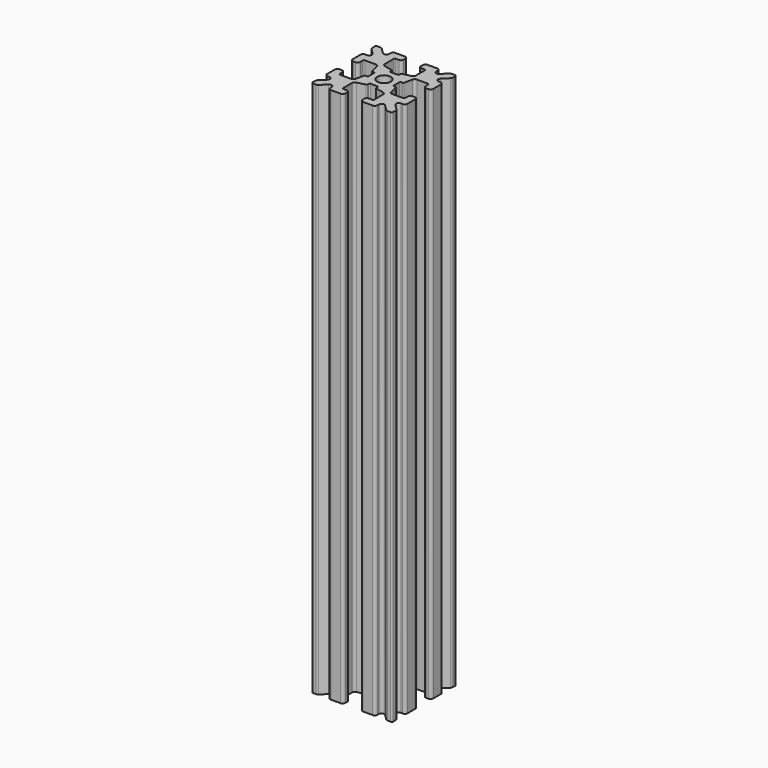
from build123d import *

# Parameters (mm, degrees)
F0_R     = 1.25
F1_DEPTH = 100


# Not quite as in the source:
# - ends of sketch curves that miss each other by under 0.0002 mm in the source are joined


with BuildPart() as f1:
    # F0 (on Top) → F1 (new body)
    with BuildSketch(Plane.XY):
        with BuildLine():
            Line((-0.6255, -2.347065), (0.6255, -2.347065))
            ThreePointArc((0.6255, -2.347065), (0.7669213562, -2.4056436438), (0.8255, -2.547065))
            Line((0.8255, -2.547065), (0.8255, -2.774891))
            ThreePointArc((0.8255, -2.774891), (0.8693776134, -2.8998942016), (0.9817580041, -2.9700489816))
            Line((0.9817580041, -2.9700489816), (2.509356, -3.312442))
            ThreePointArc((2.509356, -3.312442), (2.7903062714, -3.4878293768), (2.9, -3.800337))
            Line((2.9, -3.800337), (2.9, -5.9))
            ThreePointArc((2.9, -5.9), (2.8414213562, -6.0414213562), (2.7, -6.1))
            Line((2.7, -6.1), (2.1, -6.1))
            ThreePointArc((2.1, -6.1), (1.7464466094, -6.2464466094), (1.6, -6.6))
            Line((1.6, -6.6), (1.6, -7))
            ThreePointArc((1.6, -7), (1.7464466094, -7.3535533906), (2.1, -7.5))
            Line((2.1, -7.5), (3.9, -7.5))
            ThreePointArc((3.9, -7.5), (4.2535533906, -7.3535533906), (4.4, -7))
            Line((4.4, -7), (4.4, -6.667767))
            ThreePointArc((4.4, -6.667767), (4.7086582838, -6.2058272337), (5.2535533906, -6.3142136094))
            Line((5.2535533906, -6.3142136094), (6.292893, -7.353553))
            ThreePointArc((6.292893, -7.353553), (6.4551049572, -7.461939631), (6.646447, -7.5))
            Line((6.646447, -7.5), (7.25, -7.5))
            ThreePointArc((7.25, -7.5), (7.4267766953, -7.4267766953), (7.5, -7.25))
            Line((7.5, -7.25), (7.5, -6.646447))
            ThreePointArc((7.5, -6.646447), (7.461939631, -6.4551049572), (7.3535528906, -6.2928931094))
            Line((7.3535528906, -6.2928931094), (6.314214, -5.253553))
            ThreePointArc((6.314214, -5.253553), (6.2058272337, -4.7086582838), (6.667767, -4.4))
            Line((6.667767, -4.4), (7, -4.4))
            ThreePointArc((7, -4.4), (7.3535533906, -4.2535533906), (7.5, -3.9))
            Line((7.5, -3.9), (7.5, -2.1))
            ThreePointArc((7.5, -2.1), (7.3535533906, -1.7464466094), (7, -1.6))
            Line((7, -1.6), (6.6, -1.6))
            ThreePointArc((6.6, -1.6), (6.2464466094, -1.7464466094), (6.1, -2.1))
            Line((6.1, -2.1), (6.1, -2.7))
            ThreePointArc((6.1, -2.7), (6.0414213562, -2.8414213562), (5.9, -2.9))
            Line((5.9, -2.9), (3.800337, -2.9))
            ThreePointArc((3.800337, -2.9), (3.4878293768, -2.7903062714), (3.3124422593, -2.5093559419))
            Line((3.3124422593, -2.5093559419), (2.970049, -0.981758))
            ThreePointArc((2.970049, -0.981758), (2.8998942016, -0.8693776134), (2.774891, -0.8255))
            Line((2.774891, -0.8255), (2.547065, -0.8255))
            ThreePointArc((2.547065, -0.8255), (2.4056436438, -0.7669213562), (2.347065, -0.6255))
            Line((2.347065, -0.6255), (2.347065, 0.6255))
            ThreePointArc((2.347065, 0.6255), (2.4056436438, 0.7669213562), (2.547065, 0.8255))
            Line((2.547065, 0.8255), (2.774891, 0.8255))
            ThreePointArc((2.774891, 0.8255), (2.8998942016, 0.8693776134), (2.9700489816, 0.9817580041))
            Line((2.9700489816, 0.9817580041), (3.312442, 2.509356))
            ThreePointArc((3.312442, 2.509356), (3.4878293768, 2.7903062714), (3.800337, 2.9))
            Line((3.800337, 2.9), (5.9, 2.9))
            ThreePointArc((5.9, 2.9), (6.0414213562, 2.8414213562), (6.1, 2.7))
            Line((6.1, 2.7), (6.1, 2.1))
            ThreePointArc((6.1, 2.1), (6.2464466094, 1.7464466094), (6.6, 1.6))
            Line((6.6, 1.6), (7, 1.6))
            ThreePointArc((7, 1.6), (7.3535533906, 1.7464466094), (7.5, 2.1))
            Line((7.5, 2.1), (7.5, 3.9))
            ThreePointArc((7.5, 3.9), (7.3535533906, 4.2535533906), (7, 4.4))
            Line((7, 4.4), (6.667767, 4.4))
            ThreePointArc((6.667767, 4.4), (6.2058272337, 4.7086582838), (6.3142136094, 5.2535533906))
            Line((6.3142136094, 5.2535533906), (7.353553, 6.292893))
            ThreePointArc((7.353553, 6.292893), (7.461939631, 6.4551049572), (7.5, 6.646447))
            Line((7.5, 6.646447), (7.5, 7.25))
            ThreePointArc((7.5, 7.25), (7.4267766953, 7.4267766953), (7.25, 7.5))
            Line((7.25, 7.5), (6.646447, 7.5))
            ThreePointArc((6.646447, 7.5), (6.4551049572, 7.461939631), (6.2928931094, 7.3535528906))
            Line((6.2928931094, 7.3535528906), (5.253553, 6.314214))
            ThreePointArc((5.253553, 6.314214), (4.7086582838, 6.2058272337), (4.4, 6.667767))
            Line((4.4, 6.667767), (4.4, 7))
            ThreePointArc((4.4, 7), (4.2535533906, 7.3535533906), (3.9, 7.5))
            Line((3.9, 7.5), (2.1, 7.5))
            ThreePointArc((2.1, 7.5), (1.7464466094, 7.3535533906), (1.6, 7))
            Line((1.6, 7), (1.6, 6.6))
            ThreePointArc((1.6, 6.6), (1.7464466094, 6.2464466094), (2.1, 6.1))
            Line((2.1, 6.1), (2.7, 6.1))
            ThreePointArc((2.7, 6.1), (2.8414213562, 6.0414213562), (2.9, 5.9))
            Line((2.9, 5.9), (2.9, 3.800337))
            ThreePointArc((2.9, 3.800337), (2.7903062714, 3.4878293768), (2.5093559419, 3.3124422593))
            Line((2.5093559419, 3.3124422593), (0.981758, 2.970049))
            ThreePointArc((0.981758, 2.970049), (0.8693776134, 2.8998942016), (0.8255, 2.774891))
            Line((0.8255, 2.774891), (0.8255, 2.547065))
            ThreePointArc((0.8255, 2.547065), (0.7669213562, 2.4056436438), (0.6255, 2.347065))
            Line((0.6255, 2.347065), (-0.6255, 2.347065))
            ThreePointArc((-0.6255, 2.347065), (-0.7669213562, 2.4056436438), (-0.8255, 2.547065))
            Line((-0.8255, 2.547065), (-0.8255, 2.774891))
            ThreePointArc((-0.8255, 2.774891), (-0.8693776134, 2.8998942016), (-0.9817580041, 2.9700489816))
            Line((-0.9817580041, 2.9700489816), (-2.509356, 3.312442))
            ThreePointArc((-2.509356, 3.312442), (-2.7903062714, 3.4878293768), (-2.9, 3.800337))
            Line((-2.9, 3.800337), (-2.9, 5.9))
            ThreePointArc((-2.9, 5.9), (-2.8414213562, 6.0414213562), (-2.7, 6.1))
            Line((-2.7, 6.1), (-2.1, 6.1))
            ThreePointArc((-2.1, 6.1), (-1.7464466094, 6.2464466094), (-1.6, 6.6))
            Line((-1.6, 6.6), (-1.6, 7))
            ThreePointArc((-1.6, 7), (-1.7464466094, 7.3535533906), (-2.1, 7.5))
            Line((-2.1, 7.5), (-3.9, 7.5))
            ThreePointArc((-3.9, 7.5), (-4.2535533906, 7.3535533906), (-4.4, 7))
            Line((-4.4, 7), (-4.4, 6.667767))
            ThreePointArc((-4.4, 6.667767), (-4.7086582838, 6.2058272337), (-5.2535533906, 6.3142136094))
            Line((-5.2535533906, 6.3142136094), (-6.292893, 7.353553))
            ThreePointArc((-6.292893, 7.353553), (-6.4551049572, 7.461939631), (-6.646447, 7.5))
            Line((-6.646447, 7.5), (-7.25, 7.5))
            ThreePointArc((-7.25, 7.5), (-7.4267766953, 7.4267766953), (-7.5, 7.25))
            Line((-7.5, 7.25), (-7.5, 6.646447))
            ThreePointArc((-7.5, 6.646447), (-7.461939631, 6.4551049572), (-7.3535528906, 6.2928931094))
            Line((-7.3535528906, 6.2928931094), (-6.314214, 5.253553))
            ThreePointArc((-6.314214, 5.253553), (-6.2058272337, 4.7086582838), (-6.667767, 4.4))
            Line((-6.667767, 4.4), (-7, 4.4))
            ThreePointArc((-7, 4.4), (-7.3535533906, 4.2535533906), (-7.5, 3.9))
            Line((-7.5, 3.9), (-7.5, 2.1))
            ThreePointArc((-7.5, 2.1), (-7.3535533906, 1.7464466094), (-7, 1.6))
            Line((-7, 1.6), (-6.6, 1.6))
            ThreePointArc((-6.6, 1.6), (-6.2464466094, 1.7464466094), (-6.1, 2.1))
            Line((-6.1, 2.1), (-6.1, 2.7))
            ThreePointArc((-6.1, 2.7), (-6.0414213562, 2.8414213562), (-5.9, 2.9))
            Line((-5.9, 2.9), (-3.800337, 2.9))
            ThreePointArc((-3.800337, 2.9), (-3.4878293768, 2.7903062714), (-3.3124422593, 2.5093559419))
            Line((-3.3124422593, 2.5093559419), (-2.970049, 0.981758))
            ThreePointArc((-2.970049, 0.981758), (-2.8998942016, 0.8693776134), (-2.774891, 0.8255))
            Line((-2.774891, 0.8255), (-2.547065, 0.8255))
            ThreePointArc((-2.547065, 0.8255), (-2.4056436438, 0.7669213562), (-2.347065, 0.6255))
            Line((-2.347065, 0.6255), (-2.347065, -0.6255))
            ThreePointArc((-2.347065, -0.6255), (-2.4056436438, -0.7669213562), (-2.547065, -0.8255))
            Line((-2.547065, -0.8255), (-2.774891, -0.8255))
            ThreePointArc((-2.774891, -0.8255), (-2.8998942016, -0.8693776134), (-2.9700489816, -0.9817580041))
            Line((-2.9700489816, -0.9817580041), (-3.312442, -2.509356))
            ThreePointArc((-3.312442, -2.509356), (-3.4878293768, -2.7903062714), (-3.800337, -2.9))
            Line((-3.800337, -2.9), (-5.9, -2.9))
            ThreePointArc((-5.9, -2.9), (-6.0414213562, -2.8414213562), (-6.1, -2.7))
            Line((-6.1, -2.7), (-6.1, -2.1))
            ThreePointArc((-6.1, -2.1), (-6.2464466094, -1.7464466094), (-6.6, -1.6))
            Line((-6.6, -1.6), (-7, -1.6))
            ThreePointArc((-7, -1.6), (-7.3535533906, -1.7464466094), (-7.5, -2.1))
            Line((-7.5, -2.1), (-7.5, -3.9))
            ThreePointArc((-7.5, -3.9), (-7.3535533906, -4.2535533906), (-7, -4.4))
            Line((-7, -4.4), (-6.667767, -4.4))
            ThreePointArc((-6.667767, -4.4), (-6.2058272337, -4.7086582838), (-6.3142136094, -5.2535533906))
            Line((-6.3142136094, -5.2535533906), (-7.353553, -6.292893))
            ThreePointArc((-7.353553, -6.292893), (-7.461939631, -6.4551049572), (-7.5, -6.646447))
            Line((-7.5, -6.646447), (-7.5, -7.25))
            ThreePointArc((-7.5, -7.25), (-7.4267766953, -7.4267766953), (-7.25, -7.5))
            Line((-7.25, -7.5), (-6.646447, -7.5))
            ThreePointArc((-6.646447, -7.5), (-6.4551049572, -7.461939631), (-6.2928931094, -7.3535528906))
            Line((-6.2928931094, -7.3535528906), (-5.253553, -6.314214))
            ThreePointArc((-5.253553, -6.314214), (-4.7086582838, -6.2058272337), (-4.4, -6.667767))
            Line((-4.4, -6.667767), (-4.4, -7))
            ThreePointArc((-4.4, -7), (-4.2535533906, -7.3535533906), (-3.9, -7.5))
            Line((-3.9, -7.5), (-2.1, -7.5))
            ThreePointArc((-2.1, -7.5), (-1.7464466094, -7.3535533906), (-1.6, -7))
            Line((-1.6, -7), (-1.6, -6.6))
            ThreePointArc((-1.6, -6.6), (-1.7464466094, -6.2464466094), (-2.1, -6.1))
            Line((-2.1, -6.1), (-2.7, -6.1))
            ThreePointArc((-2.7, -6.1), (-2.8414213562, -6.0414213562), (-2.9, -5.9))
            Line((-2.9, -5.9), (-2.9, -3.800337))
            ThreePointArc((-2.9, -3.800337), (-2.7903062714, -3.4878293768), (-2.5093559419, -3.3124422593))
            Line((-2.5093559419, -3.3124422593), (-0.981758, -2.970049))
            ThreePointArc((-0.981758, -2.970049), (-0.8693776134, -2.8998942016), (-0.8255, -2.774891))
            Line((-0.8255, -2.774891), (-0.8255, -2.547065))
            ThreePointArc((-0.8255, -2.547065), (-0.7669213562, -2.4056436438), (-0.6255, -2.347065))
        make_face()
        Circle(F0_R, mode=Mode.SUBTRACT)
    extrude(amount=F1_DEPTH)


solid = f1.part
